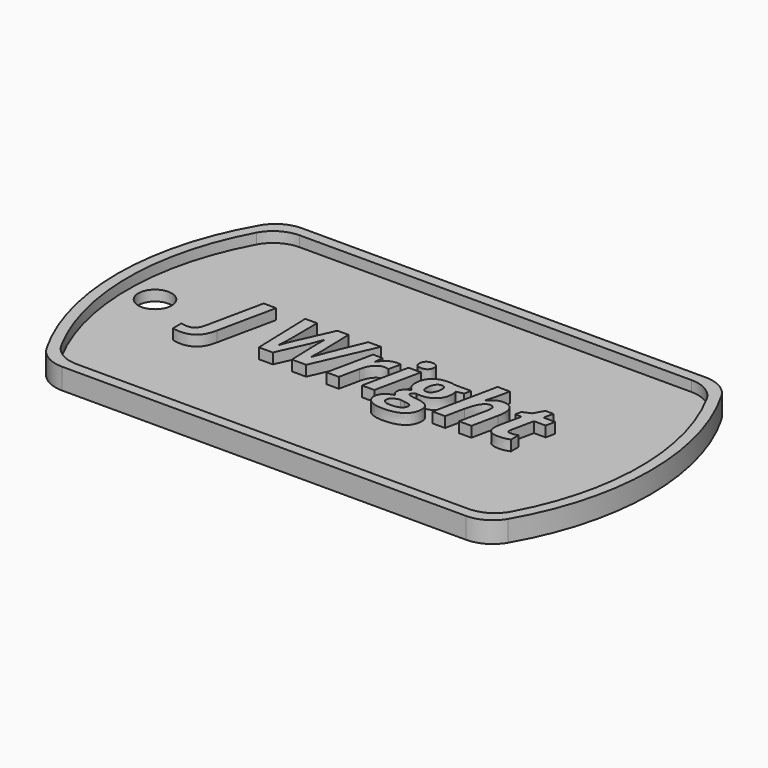
from build123d import *

# Parameters (mm, degrees)
F1_DEPTH     = 1
F3_DEPTH     = 1
F4_R         = 1.5875
F5_DEPTH     = 1
F6_TEXT_SIZE = 8.0415663736
F7_DEPTH     = 1


# Not quite as in the source:
# - Text() gives the source's letters only with a copy of the font that has no kerning and outlines rounded to 1/6400 em; it was checked with that copy


with BuildPart() as f1:
    # F0 (on Top) → F1 (new body)
    with BuildSketch(Plane.XY):
        with BuildLine():
            ThreePointArc((-19.2474145991, 14.2875), (-20.8349145991, 13.862130657), (-21.9970452561, 12.7))
            ThreePointArc((-21.9970452561, 12.7), (-25.4, 0), (-21.9970452561, -12.7))
            ThreePointArc((-21.9970452561, -12.7), (-20.8349145991, -13.862130657), (-19.2474145991, -14.2875))
            Line((-19.2474145991, -14.2875), (19.2474145991, -14.2875))
            ThreePointArc((19.2474145991, -14.2875), (20.8349145991, -13.862130657), (21.9970452561, -12.7))
            ThreePointArc((21.9970452561, -12.7), (25.4, 0), (21.9970452561, 12.7))
            ThreePointArc((21.9970452561, 12.7), (20.8349145991, 13.862130657), (19.2474145991, 14.2875))
            Line((19.2474145991, 14.2875), (-19.2474145991, 14.2875))
        make_face()
    extrude(amount=F1_DEPTH)

    # F2 (on face) → F3 (join)
    with BuildSketch(Plane.XY.offset(1)):
        with BuildLine():
            Line((19.2474145991, 14.2875), (-19.2474145991, 14.2875))
            ThreePointArc((-19.2474145991, 14.2875), (-20.8349145991, 13.862130657), (-21.9970452561, 12.7))
            ThreePointArc((-21.9970452561, 12.7), (-25.4, 0), (-21.9970452561, -12.7))
            ThreePointArc((-21.9970452561, -12.7), (-20.8349145991, -13.862130657), (-19.2474145991, -14.2875))
            Line((-19.2474145991, -14.2875), (19.2474145991, -14.2875))
            ThreePointArc((19.2474145991, -14.2875), (20.8349145991, -13.862130657), (21.9970452561, -12.7))
            ThreePointArc((21.9970452561, -12.7), (25.4, 0), (21.9970452561, 12.7))
            ThreePointArc((21.9970452561, 12.7), (20.8349145991, 13.862130657), (19.2474145991, 14.2875))
        make_face()
        with BuildLine():
            ThreePointArc((-21.4526124879, 11.6252061249), (-20.2856017842, 12.8404540819), (-18.6611352482, 13.2875))
            Line((-18.6611352482, 13.2875), (18.6611352482, 13.2875))
            ThreePointArc((18.6611352482, 13.2875), (20.2856017842, 12.8404540819), (21.4526124879, 11.6252061249))
            ThreePointArc((21.4526124879, 11.6252061249), (24.4, 0), (21.4526124879, -11.6252061249))
            ThreePointArc((21.4526124879, -11.6252061249), (20.2856017842, -12.8404540819), (18.6611352482, -13.2875))
            Line((18.6611352482, -13.2875), (-18.6611352482, -13.2875))
            ThreePointArc((-18.6611352482, -13.2875), (-20.2856017842, -12.8404540819), (-21.4526124879, -11.6252061249))
            ThreePointArc((-21.4526124879, -11.6252061249), (-24.4, 0), (-21.4526124879, 11.6252061249))
        make_face(mode=Mode.SUBTRACT)
    extrude(amount=F3_DEPTH)

    # F4 (on face) → F5 (cut)
    with BuildSketch(Plane.XY.offset(1)):
        with Locations((-21.821282804, 0)):
            Circle(F4_R)
    extrude(amount=-F5_DEPTH, mode=Mode.SUBTRACT)

    # F6 (on face) → F7 (join)
    with BuildSketch(Plane.XY.offset(1)):
        with Locations((-15.4122849926, -2.7017042739)):
            Text('J Wright', F6_TEXT_SIZE, font='Open Sans', font_style=FontStyle.BOLDITALIC, text_align=(TextAlign.LEFT, TextAlign.BOTTOM))
    extrude(amount=F7_DEPTH)


solid = f1.part
